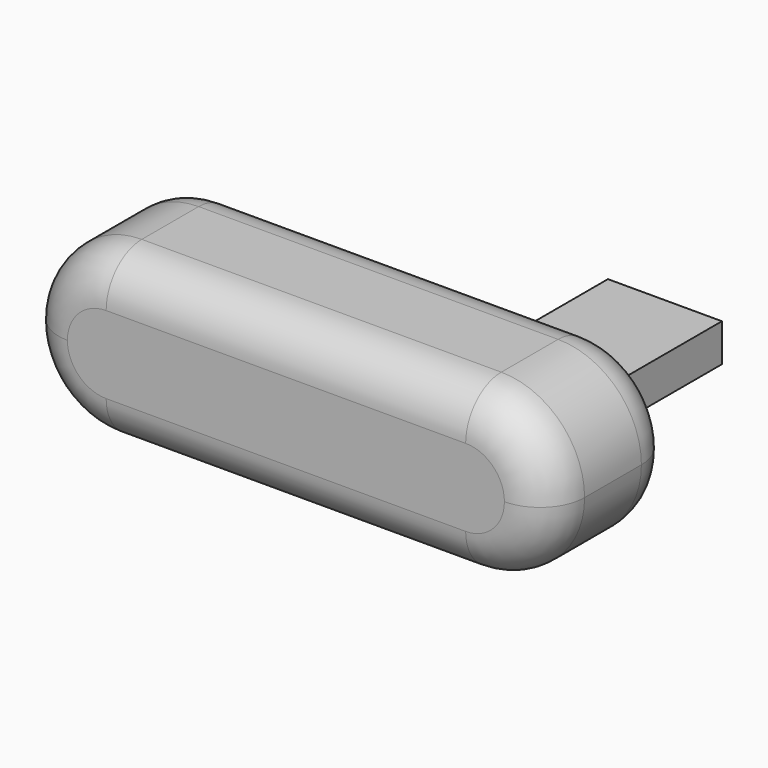
from build123d import *

# Parameters (mm, degrees)
F0_W     = 60
F0_H     = 19
F1_DEPTH = 9.13
F2_R     = 9.49999
F3_W     = 13
F3_H     = 4.318
F4_DEPTH = 19.05
F5_SIZE  = 1.27
F6_R     = 5.08


# Not quite as in the source:
# - a fillet or chamfer is up to 0.001 mm smaller than in the source, because OpenCascade refuses the exact size


with BuildPart() as f1:
    # F0 (on Front) → F1 (new body, symmetric)
    with BuildSketch(Plane.XZ):
        Rectangle(F0_W, F0_H)
    extrude(amount=F1_DEPTH, both=True)

    # F2 (radius 9.5 in the source; OpenCascade refuses exactly that, so slightly less here)
    f2_edges = [f1.edges().sort_by_distance(p)[0] for p in [
        (30, 0, 9.5),
        (30, 0, -9.5),
        (-30, 0, 9.5),
        (-30, 0, -9.5),
    ]]
    fillet(f2_edges, radius=F2_R)

    # F3 (on face) → F4 (join)
    with BuildSketch(Plane(origin=(0, 9.13, 0), x_dir=(-1, 0, 0), z_dir=(0, 1, 0))):
        with Locations((-14.3949933554, 0)):
            Rectangle(F3_W, F3_H)
    extrude(amount=F4_DEPTH)

    # F5
    f5_edges = [f1.edges().sort_by_distance(p)[0] for p in [
        (14.394993, 28.18, 2.159),
        (20.894993, 28.18, 0),
        (7.894993, 28.18, 0),
        (14.394993, 28.18, -2.159),
    ]]
    chamfer(f5_edges, length=F5_SIZE)

    # F6
    f6_edges = [f1.edges().sort_by_distance(p)[0] for p in [
        (0, 9.13, 9.5),
        (0, -9.13, 9.5),
    ]]
    fillet(f6_edges, radius=F6_R)


solid = f1.part
